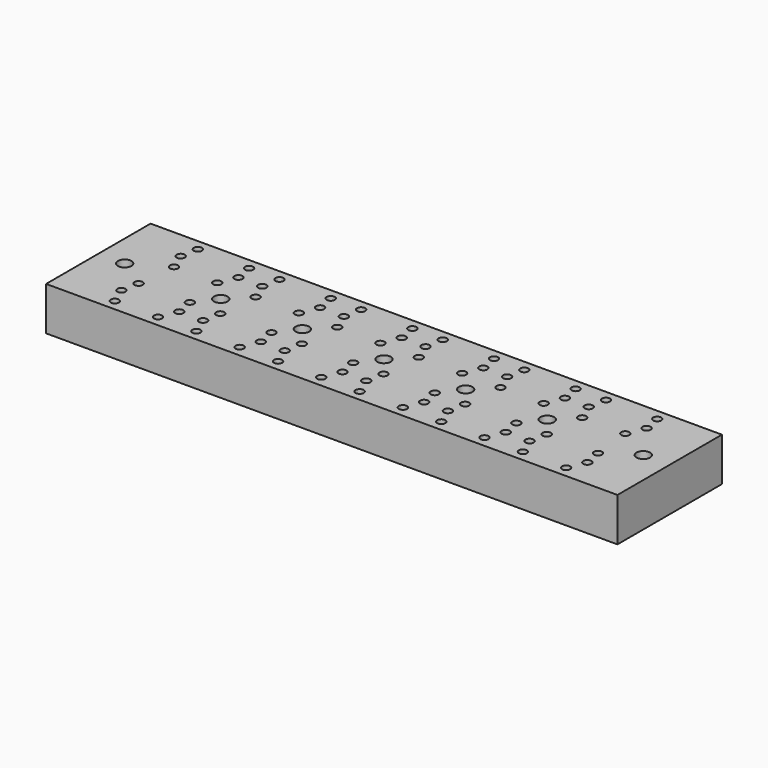
from build123d import *

# Parameters (mm, degrees)
F0_W     = 333.375
F0_H     = 76.2
F1_DEPTH = 25.4
F2_D     = 7.9375
F2_DEPTH = 50.8
F2_TIP   = 2.3846655818
F3_D     = 4.7625
F3_DEPTH = 25.4
F3_TIP   = 1.4307993491
F5_D     = 4.7625
F5_DEPTH = 25.4
F5_TIP   = 1.4307993491


# Not quite as in the source:
# - a feature names something its author has since deleted; it is built from what else it names


with BuildPart() as f1:
    # F0 (on Top) → F1 (new body)
    with BuildSketch(Plane.XY):
        with Locations((166.6875, 38.1)):
            Rectangle(F0_W, F0_H)
    extrude(amount=F1_DEPTH)

    # F2
    with Locations(Plane(origin=(0, 0, 0), x_dir=(1, 0, 0), z_dir=(0, 0, -1))):
        with Locations((15.382875, -38.1), (71.4375, -38.1), (119.0625, -38.1), (166.6875, -38.1), (214.3125, -38.1), (261.9375, -38.1), (317.992125, -38.1)):
            Hole(F2_D / 2, depth=F2_DEPTH)
            with Locations((0, 0, -(F2_DEPTH + F2_TIP / 2))):  # 118° drill point
                Cone(0, F2_D / 2, F2_TIP, mode=Mode.SUBTRACT)

    # F3
    with Locations(Plane(origin=(0, 0, 0), x_dir=(1, 0, 0), z_dir=(0, 0, -1))):
        with Locations((30.76575, -16.51), (64.48425, -16.51), (78.39075, -16.51), (112.10925, -16.51), (126.01575, -16.51), (30.76575, -59.69), (64.48425, -59.69), (78.39075, -59.69), (112.10925, -59.69), (126.01575, -59.69), (159.73425, -59.69), (173.64075, -59.69), (159.73425, -16.51), (173.64075, -16.51), (207.35925, -16.51), (221.26575, -16.51), (254.98425, -16.51), (268.89075, -16.51), (302.60925, -16.51), (207.35925, -59.69), (221.26575, -59.69), (254.98425, -59.69), (268.89075, -59.69), (302.60925, -59.69)):
            Hole(F3_D / 2, depth=F3_DEPTH)
            with Locations((0, 0, -(F3_DEPTH + F3_TIP / 2))):  # 118° drill point
                Cone(0, F3_D / 2, F3_TIP, mode=Mode.SUBTRACT)

    # F5
    with Locations(Plane.XY.offset(25.4)):
        with Locations((32.67075, 69.85), (35.02025, 49.53), (62.57925, 69.85), (60.22975, 49.53), (80.29575, 69.85), (82.64525, 49.53), (110.20425, 69.85), (107.85475, 49.53), (127.92075, 69.85), (130.27025, 49.53), (157.82925, 69.85), (155.47975, 49.53), (175.54575, 69.85), (177.89525, 49.53), (205.45425, 69.85), (203.10475, 49.53), (223.17075, 69.85), (225.52025, 49.53), (253.07925, 69.85), (250.72975, 49.53), (270.79575, 69.85), (273.14525, 49.53), (300.70425, 69.85), (298.35475, 49.53), (32.67075, 26.67), (35.02025, 6.35), (62.57925, 26.67), (60.22975, 6.35), (80.29575, 26.67), (82.64525, 6.35), (110.20425, 26.67), (107.85475, 6.35), (127.92075, 26.67), (130.27025, 6.35), (157.82925, 26.67), (155.47975, 6.35), (175.54575, 26.67), (177.89525, 6.35), (205.45425, 26.67), (203.10475, 6.35), (223.17075, 26.67), (225.52025, 6.35), (253.07925, 26.67), (250.72975, 6.35), (270.79575, 26.67), (273.14525, 6.35), (300.70425, 26.67), (298.35475, 6.35)):
            Hole(F5_D / 2, depth=F5_DEPTH)
            with Locations((0, 0, -(F5_DEPTH + F5_TIP / 2))):  # 118° drill point
                Cone(0, F5_D / 2, F5_TIP, mode=Mode.SUBTRACT)


solid = f1.part
